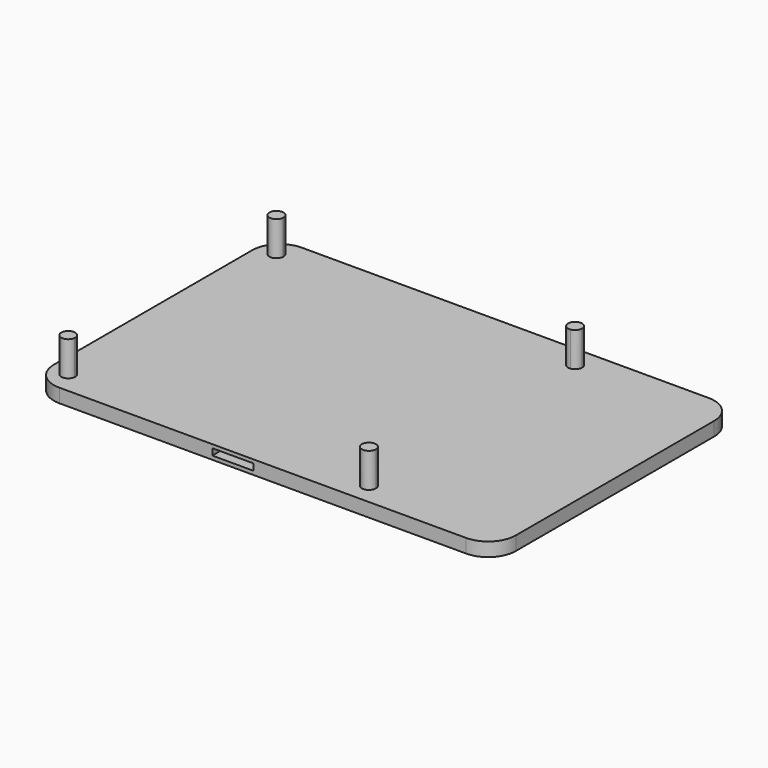
from build123d import *

# Parameters (mm, degrees)
F1_DEPTH = 2.54
F2_R     = 5.08
F3_DEPTH = 8.89
F5_W     = 7.6071470976
F5_H     = 1.2031628285
F6_DEPTH = 4.318
F7_W     = 7.584489882
F7_H     = 1.1869876339
F8_DEPTH = 4.318


# Not quite as in the source:
# - ends of sketch curves that miss each other by under 0.0002 mm in the source are joined


with BuildPart() as f1:
    # F0 (on Top) → F1 (new body)
    with BuildSketch(Plane.XY):
        with BuildLine():
            Line((-42.6210959934, 27.9657971114), (-42.6210959934, 24.0334319246))
            Line((-42.6210959934, 24.0334319246), (-40.4223592815, 24.0334319246))
            ThreePointArc((-40.4223592815, 24.0334319246), (-39.1720464715, 25.4046969243), (-37.8398531152, 24.1128336638))
            ThreePointArc((-37.8398531152, 24.1128336638), (-37.8404635808, 24.0731140337), (-37.8422944012, 24.0334319246))
            Line((-37.8422944012, 24.0334319246), (14.8014883525, 24.0334319246))
            ThreePointArc((14.8014883525, 24.0334319246), (16.1318254594, 25.2445390274), (17.3839117365, 23.9526964724))
            ThreePointArc((17.3839117365, 23.9526964724), (17.080387221, 23.1205499759), (16.312373062, 22.6792460274))
            Line((16.312373062, 22.6792460274), (16.4525141181, -22.7324364705))
            ThreePointArc((16.4525141181, -22.7324364705), (17.3541679288, -23.1175729008), (17.726055436, -24.0247715265))
            ThreePointArc((17.726055436, -24.0247715265), (17.7260481822, -24.0291017499), (17.7260264206, -24.0334319246))
            Line((17.7260264206, -24.0334319246), (42.6210959934, -24.0334319246))
            Line((42.6210959934, -24.0334319246), (42.6210959934, 24.0334319246))
            Line((42.6210959934, 24.0334319246), (42.6210959934, 27.965891646))
            Line((42.6210959934, 27.965891646), (-42.6210959934, 27.9657971114))
        make_face()
        with BuildLine():
            Line((-42.6210959934, 24.0334319246), (-42.6210959934, -24.0334319246))
            Line((-42.6210959934, -24.0334319246), (-40.4303500829, -24.0334319246))
            ThreePointArc((-40.4303500829, -24.0334319246), (-39.2142367954, -22.6050090303), (-37.8527686966, -23.8956399262))
            ThreePointArc((-37.8527686966, -23.8956399262), (-37.8546115269, -23.9646342987), (-37.8601347627, -24.0334319246))
            Line((-37.8601347627, -24.0334319246), (15.1411369991, -24.0334319246))
            ThreePointArc((15.1411369991, -24.0334319246), (15.5233039011, -23.1072298959), (16.4525141181, -22.7324364705))
            Line((16.4525141181, -22.7324364705), (16.312373062, 22.6792460274))
            ThreePointArc((16.312373062, 22.6792460274), (15.2287950262, 22.9902332706), (14.8014883525, 24.0334319246))
            Line((14.8014883525, 24.0334319246), (-37.8422944012, 24.0334319246))
            ThreePointArc((-37.8422944012, 24.0334319246), (-39.1323268414, 22.8203599376), (-40.4223592815, 24.0334319246))
            Line((-40.4223592815, 24.0334319246), (-42.6210959934, 24.0334319246))
        make_face()
        with BuildLine():
            Line((-40.4303500829, -24.0334319246), (-42.6210959934, -24.0334319246))
            Line((-42.6210959934, -24.0334319246), (-42.6210959934, -27.965891646))
            Line((-42.6210959934, -27.965891646), (42.6210959934, -27.965891646))
            Line((42.6210959934, -27.965891646), (42.6210959934, -24.0334319246))
            Line((42.6210959934, -24.0334319246), (17.7260264206, -24.0334319246))
            ThreePointArc((17.7260264206, -24.0334319246), (16.4335817099, -25.3172452526), (15.1411369991, -24.0334319246))
            Line((15.1411369991, -24.0334319246), (-37.8601347627, -24.0334319246))
            ThreePointArc((-37.8601347627, -24.0334319246), (-39.1452424228, -25.1881136524), (-40.4303500829, -24.0334319246))
        make_face()
    extrude(amount=F1_DEPTH)

    # F2
    f2_edges = [f1.edges().sort_by_distance(p)[0] for p in [
        (42.621096, -27.965892, 1.27),
        (-42.621096, -27.965892, 1.27),
        (42.621096, 27.965892, 1.27),
        (-42.621096, 27.965797, 1.27),
    ]]
    fillet(f2_edges, radius=F2_R)

    # F0 (on Top) → F3 (join)
    with BuildSketch(Plane.XY):
        with BuildLine():
            ThreePointArc((-37.8398531152, 24.1128336638), (-39.1720464715, 25.4046969243), (-40.4223592815, 24.0334319246))
            Line((-40.4223592815, 24.0334319246), (-37.8422944012, 24.0334319246))
            ThreePointArc((-37.8422944012, 24.0334319246), (-37.8404635808, 24.0731140337), (-37.8398531152, 24.1128336638))
        make_face()
        with BuildLine():
            Line((-37.8422944012, 24.0334319246), (-40.4223592815, 24.0334319246))
            ThreePointArc((-40.4223592815, 24.0334319246), (-39.1323268414, 22.8203599376), (-37.8422944012, 24.0334319246))
        make_face()
        with BuildLine():
            ThreePointArc((-37.8527686966, -23.8956399262), (-39.2142367954, -22.6050090303), (-40.4303500829, -24.0334319246))
            Line((-40.4303500829, -24.0334319246), (-37.8601347627, -24.0334319246))
            ThreePointArc((-37.8601347627, -24.0334319246), (-37.8546115269, -23.9646342987), (-37.8527686966, -23.8956399262))
        make_face()
        with BuildLine():
            Line((-37.8601347627, -24.0334319246), (-40.4303500829, -24.0334319246))
            ThreePointArc((-40.4303500829, -24.0334319246), (-39.1452424228, -25.1881136524), (-37.8601347627, -24.0334319246))
        make_face()
        with BuildLine():
            ThreePointArc((17.3839117365, 23.9526964724), (16.1318254594, 25.2445390274), (14.8014883525, 24.0334319246))
            Line((14.8014883525, 24.0334319246), (16.3081940264, 24.0334319246))
            Line((16.3081940264, 24.0334319246), (16.312373062, 22.6792460274))
            ThreePointArc((16.312373062, 22.6792460274), (17.080387221, 23.1205499759), (17.3839117365, 23.9526964724))
        make_face()
        with BuildLine():
            Line((16.3081940264, 24.0334319246), (14.8014883525, 24.0334319246))
            ThreePointArc((14.8014883525, 24.0334319246), (15.2287950262, 22.9902332706), (16.312373062, 22.6792460274))
            Line((16.312373062, 22.6792460274), (16.3081940264, 24.0334319246))
        make_face()
        with BuildLine():
            Line((16.4525141181, -22.7324364705), (16.4565290074, -24.0334319246))
            Line((16.4565290074, -24.0334319246), (17.7260264206, -24.0334319246))
            ThreePointArc((17.7260264206, -24.0334319246), (17.7260481822, -24.0291017499), (17.726055436, -24.0247715265))
            ThreePointArc((17.726055436, -24.0247715265), (17.3541679288, -23.1175729008), (16.4525141181, -22.7324364705))
        make_face()
        with BuildLine():
            ThreePointArc((16.4525141181, -22.7324364705), (15.5233039011, -23.1072298959), (15.1411369991, -24.0334319246))
            Line((15.1411369991, -24.0334319246), (16.4565290074, -24.0334319246))
            Line((16.4565290074, -24.0334319246), (16.4525141181, -22.7324364705))
        make_face()
        with BuildLine():
            Line((16.4565290074, -24.0334319246), (15.1411369991, -24.0334319246))
            ThreePointArc((15.1411369991, -24.0334319246), (16.4335817099, -25.3172452526), (17.7260264206, -24.0334319246))
            Line((17.7260264206, -24.0334319246), (16.4565290074, -24.0334319246))
        make_face()
    extrude(amount=F3_DEPTH)

    # F5 (on face) → F6 (cut)
    with BuildSketch(Plane.XZ.offset(27.965891646)):
        with Locations((-5.5109024979, 1.2853431981)):
            Rectangle(F5_W, F5_H)
    extrude(amount=-F6_DEPTH, mode=Mode.SUBTRACT)

    # F7 (on face) → F8 (cut)
    with BuildSketch(Plane(origin=(0, 27.965891646, 0), x_dir=(-1, 0, 0), z_dir=(0, 1, 0))):
        with Locations((31.9627784193, 1.27)):
            Rectangle(F7_W, F7_H)
    extrude(amount=-F8_DEPTH, mode=Mode.SUBTRACT)


solid = f1.part
